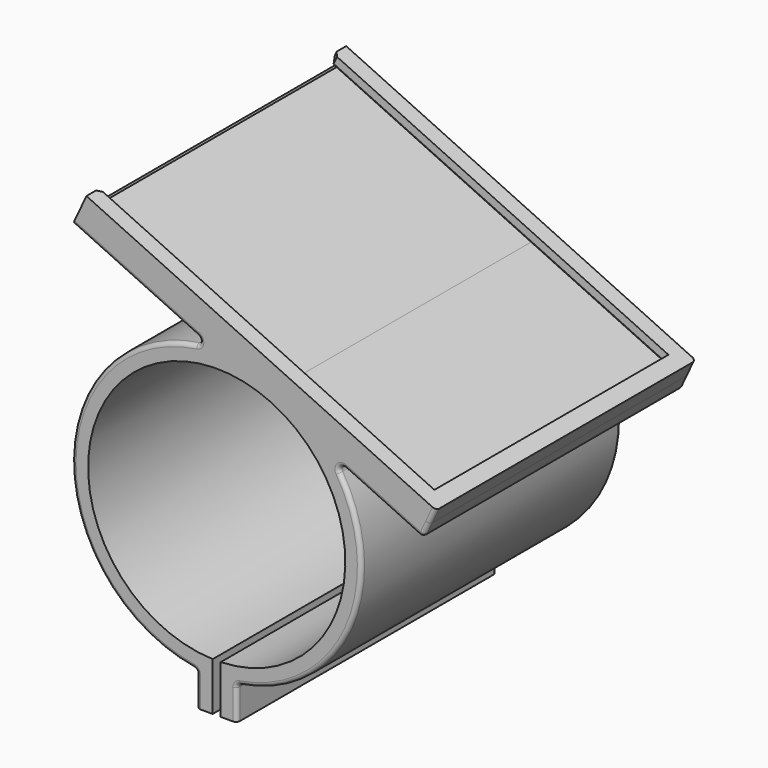
from build123d import *

# Parameters (mm, degrees)
F1_DEPTH     = 64.135
F3_DEPTH     = 76.2
F5_DEPTH     = 3.175
F6_R         = 0.79375
F7_T1_DEPTH  = 3.6287733717
F7_T6_DEPTH  = 4.4225233717
F7_T8_DEPTH  = 4.8762967434
F7_T13_DEPTH = 63.7950233717
F7_T18_DEPTH = 4.4225233717
F7_T23_DEPTH = 6.4637967434
F7_T25_DEPTH = 4.8762967434


# Not quite as in the source:
# - a fillet or chamfer that OpenCascade refuses, or shapes differently, is made with other operations: its cross-section is extruded or revolved along the edge and cut away or added


with BuildPart() as f1:
    # F0 (on Front) → F1 (new body)
    with BuildSketch(Plane.XZ):
        with BuildLine():
            ThreePointArc((10.7345036748, 23.0202178716), (24.8808005482, -5.1093800095), (0.79375, -25.3875946269))
            Line((0.79375, -25.3875946269), (0.79375, -28.563973567))
            ThreePointArc((0.79375, -28.563973567), (2.3849591955, -28.4752979727), (3.96875, -28.2980502586))
            ThreePointArc((3.96875, -28.2980502586), (26.4678099831, -10.7696638619), (22.5988525327, 17.4877811401))
            Line((22.5988525327, 17.4877811401), (10.7345036748, 23.0202178716))
        make_face()
        with BuildLine():
            Line((-1.1298448363, 28.5526544413), (10.7345036748, 23.0202178716))
            Line((10.7345036748, 23.0202178716), (22.5988525327, 17.4877811401))
            ThreePointArc((22.5988525327, 17.4877811401), (17.8402275241, 22.3216689987), (12.0763169886, 25.8977449403))
            ThreePointArc((12.0763169886, 25.8977449403), (5.6319134635, 28.0144993841), (-1.1298448363, 28.5526544413))
        make_face()
        with BuildLine():
            ThreePointArc((-0.79375, -25.3875946269), (-24.708980627, 5.8844096028), (10.7345036748, 23.0202178716))
            Line((10.7345036748, 23.0202178716), (-1.1298448363, 28.5526544413))
            ThreePointArc((-1.1298448363, 28.5526544413), (-28.5394389143, 1.4251496253), (-3.96875, -28.2980502586))
            ThreePointArc((-3.96875, -28.2980502586), (-2.3849591955, -28.4752979727), (-0.79375, -28.563973567))
            Line((-0.79375, -28.563973567), (-0.79375, -25.3875946269))
        make_face()
        with BuildLine():
            ThreePointArc((3.96875, -28.2980502586), (2.3849591955, -28.4752979727), (0.79375, -28.563973567))
            Line((0.79375, -28.563973567), (0.79375, -34.925))
            Line((0.79375, -34.925), (3.96875, -34.925))
            Line((3.96875, -34.925), (3.96875, -28.2980502586))
        make_face()
        with BuildLine():
            ThreePointArc((12.0763169886, 25.8977449403), (17.8402275241, 22.3216689987), (22.5988525327, 17.4877811401))
            Line((22.5988525327, 17.4877811401), (40.6476504402, 9.0714884554))
            Line((40.6476504402, 9.0714884554), (41.9894634213, 11.9490156792))
            Line((41.9894634213, 11.9490156792), (12.0763169886, 25.8977449403))
        make_face()
        with BuildLine():
            Line((-28.413002932, 41.275), (-1.1298448363, 28.5526544413))
            ThreePointArc((-1.1298448363, 28.5526544413), (5.6319134635, 28.0144993841), (12.0763169886, 25.8977449403))
            Line((12.0763169886, 25.8977449403), (-27.0711899509, 44.1525272238))
            Line((-27.0711899509, 44.1525272238), (-28.413002932, 41.275))
        make_face()
        with BuildLine():
            Line((-0.79375, -34.925), (-0.79375, -28.563973567))
            ThreePointArc((-0.79375, -28.563973567), (-2.3849591955, -28.4752979727), (-3.96875, -28.2980502586))
            Line((-3.96875, -28.2980502586), (-3.96875, -34.925))
            Line((-3.96875, -34.925), (-0.79375, -34.925))
        make_face()
    extrude(amount=F1_DEPTH)

    # F2 (on face) → F3 (join, through all)
    with BuildSketch(Plane(origin=(-39.1475067802, 0, 18.2547822093), x_dir=(0, -1, 0), z_dir=(-0.906307787, 0, 0.4226182617))):
        Polygon((0, 31.75), (0, 28.575), (1.5875, 28.575), (1.5875, 30.1625), (3.175, 30.1625), (3.175, 31.75), align=None)
        Polygon((62.5475, 30.1625), (62.5475, 28.575), (64.135, 28.575), (64.135, 31.75), (60.96, 31.75), (60.96, 30.1625), align=None)
    extrude(amount=-F3_DEPTH)

    # F4 (on face) → F5 (join)
    with BuildSketch(Plane(origin=(29.913146592, 0, -13.9487293354), x_dir=(0, 1, 0), z_dir=(0.906307787, 0, -0.4226182617))):
        Polygon((-3.175, 31.75), (-60.96, 31.75), (-60.96, 30.1625), (-62.5475, 30.1625), (-62.5475, 28.575), (-1.5875, 28.575), (-1.5875, 30.1625), (-3.175, 30.1625), align=None)
    extrude(amount=-F5_DEPTH)

    # F6
    f6_edges = [f1.edges().sort_by_distance(p)[0] for p in [
        (-28.539439, 0, 1.42515),
        (-28.539439, -64.135, 1.42515),
        (-1.129845, -32.0675, 28.552654),
        (-3.96875, -32.0675, -28.29805),
        (22.598853, -32.0675, 17.487781),
        (3.96875, -32.0675, -28.29805),
        (26.46781, 0, -10.769664),
        (26.46781, -64.135, -10.769664),
        (41.989463, 0, 11.949016),
        (40.64765, -32.0675, 9.071488),
        (41.989463, -64.135, 11.949016),
        (3.96875, -64.135, -31.611525),
        (31.623251, -64.135, 13.279635),
        (-14.771424, -64.135, 34.913827),
        (-3.96875, -64.135, -31.611525),
        (-3.96875, 0, -31.611525),
        (-14.771424, 0, 34.913827),
        (31.623251, 0, 13.279635),
        (3.96875, 0, -31.611525),
    ]]
    fillet(f6_edges, radius=F6_R)

    # F7: chamfer of 0.79375 on 7 edges, made by hand

    # F7_s2 → F7_t1 (cut)
    with BuildSketch(Plane.XZ.offset(1.5875)):
        Polygon((-26.0648302152, 46.3106726417), (-25.6809016545, 45.2558375905), (-26.4002834604, 45.5912908358), align=None)
    extrude(amount=F7_T1_DEPTH, mode=Mode.SUBTRACT)


with BuildPart() as f7_tool4:
    # F7_s5 → F7_t6 (new body)
    with BuildSketch(Plane(origin=(12.0763168292, 0, 25.8977450146), x_dir=(0, 1, 0), z_dir=(0.4226182617, 0, 0.906307787))):
        Polygon((-0.79375, 43.1944945637), (-1.5875, 42.4007445637), (-1.5875, 43.1944945637), align=None)
    extrude(amount=F7_T6_DEPTH)

    split(bisect_by=Plane(origin=(-8.131860996, 0, -2.9597553517), x_dir=(0, 1, 0), z_dir=(-0.9396926208, 0, -0.3420201433)), keep=Keep.TOP)


with BuildPart() as f1_1:
    add(f1.part)

    # F7_t3: cut F7_tool4
    add(f7_tool4.part, mode=Mode.SUBTRACT)

    # F7_s9 → F7_t8 (cut)
    with BuildSketch(Plane(origin=(12.2199971609, 0, 26.2058684802), x_dir=(0, 1, 0), z_dir=(0.4226182617, 0, 0.906307787))):
        Polygon((-2.38125, 43.1944945637), (-3.175, 42.4007445637), (-3.175, 43.1944945637), align=None)
    extrude(amount=F7_T8_DEPTH, mode=Mode.SUBTRACT)


with BuildPart() as f7_tool11:
    # F7_s12 → F7_t13 (new body)
    with BuildSketch(Plane.XZ.offset(62.5475)):
        Polygon((-27.4066431962, 43.4331454179), (-26.351808145, 43.8170739786), (-27.0711899509, 44.1525272238), align=None)
    extrude(amount=-F7_T13_DEPTH)

    split(bisect_by=Plane(origin=(-19.9334442931, -21.9941222818, 9.2951177273), x_dir=(0.7409656453, -0.6715429342, 0), z_dir=(-0.6408563821, -0.7071067812, 0.2988362387)), keep=Keep.TOP)


with BuildPart() as f1_2:
    add(f1_1.part)

    # F7_t10: cut F7_tool11
    add(f7_tool11.part, mode=Mode.SUBTRACT)


with BuildPart() as f7_tool16:
    # F7_s17 → F7_t18 (new body)
    with BuildSketch(Plane(origin=(12.7472233198, 0, 27.3365086265), x_dir=(0, 1, 0), z_dir=(-0.4226182617, 0, -0.906307787))):
        Polygon((-63.34125, -43.1944945637), (-62.5475, -42.4007445637), (-62.5475, -43.1944945637), align=None)
    extrude(amount=F7_T18_DEPTH)

    split(bisect_by=Plane(origin=(-17.1651120978, 0, 47.160757891), x_dir=(0, 1, 0), z_dir=(-0.3420201433, 0, 0.9396926208)), keep=Keep.TOP)


with BuildPart() as f1_3:
    add(f1_2.part)

    # F7_t15: cut F7_tool16
    add(f7_tool16.part, mode=Mode.SUBTRACT)


with BuildPart() as f7_tool21:
    # F7_s22 → F7_t23 (new body)
    with BuildSketch(Plane.XZ.offset(58.9187266283)):
        Polygon((-26.0648302152, 46.3106726417), (-25.6809016545, 45.2558375905), (-26.4002834604, 45.5912908358), align=None)
    extrude(amount=F7_T23_DEPTH)

    split(bisect_by=Plane(origin=(9.1295806677, -10.0733777182, -4.2571933811), x_dir=(-0.7409656453, -0.6715429342, 0), z_dir=(-0.6408563821, 0.7071067812, 0.2988362387)), keep=Keep.TOP)


with BuildPart() as f1_4:
    add(f1_3.part)

    # F7_t20: cut F7_tool21
    add(f7_tool21.part, mode=Mode.SUBTRACT)

    # F7_s26 → F7_t25 (cut)
    with BuildSketch(Plane(origin=(14.2808092144, 0, 30.6252941907), x_dir=(0, 1, 0), z_dir=(-0.4226182617, 0, -0.906307787))):
        Polygon((-61.75375, -43.1944945637), (-60.96, -42.4007445637), (-60.96, -43.1944945637), align=None)
    extrude(amount=F7_T25_DEPTH, mode=Mode.SUBTRACT)


solid = f1_4.part
